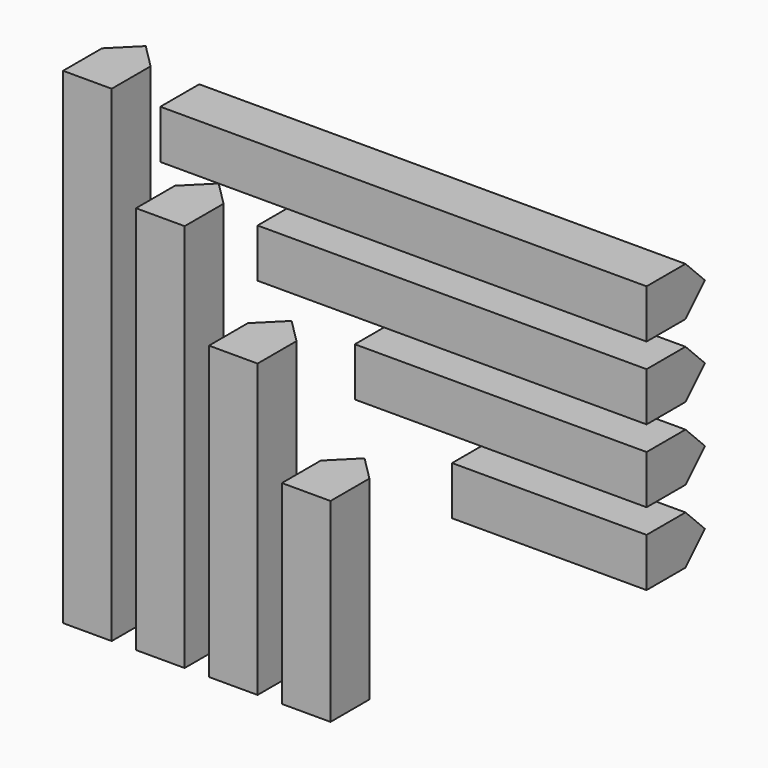
from build123d import *

# Parameters (mm, degrees)
F0_W      = 10
F0_H      = 100
F1_DEPTH  = 15
F0_H_2    = 80
F0_H_3    = 60
F0_H_4    = 40
F0_W_2    = 100
F0_H_5    = 10
F0_W_3    = 80
F0_W_4    = 60
F0_W_5    = 40
F2_SIZE   = 4.99999
F2_2_SIZE = 4.99999
F2_3_SIZE = 4.99999
F2_4_SIZE = 4.99999
F2_5_SIZE = 4.99999
F2_6_SIZE = 4.99999
F2_7_SIZE = 4.99999
F2_8_SIZE = 4.99999


# Not quite as in the source:
# - a fillet or chamfer is up to 0.001 mm smaller than in the source, because OpenCascade refuses the exact size


with BuildPart() as f1:
    # F0 (on Front) → F1 (new body)
    with BuildSketch(Plane.XZ):
        with Locations((-76.6543754238, -0.7175691426)):
            Rectangle(F0_W, F0_H)
    extrude(amount=F1_DEPTH)

    # F2#8 (size 5 in the source; OpenCascade refuses exactly that, so slightly less here)
    f2_8_edges = [f1.edges().sort_by_distance(p)[0] for p in [
        (-71.654375, 0, -0.717569),
        (-81.654375, 0, -0.717569),
    ]]
    chamfer(f2_8_edges, length=F2_8_SIZE)


with BuildPart() as f1b:
    # F0 (on Front) → F1, piece 2 (new body)
    with BuildSketch(Plane.XZ):
        with Locations((-61.6543754238, -10.7175691426)):
            Rectangle(F0_W, F0_H_2)
    extrude(amount=F1_DEPTH)

    # F2#7 (size 5 in the source; OpenCascade refuses exactly that, so slightly less here)
    f2_7_edges = [f1b.edges().sort_by_distance(p)[0] for p in [
        (-56.654375, 0, -10.717569),
        (-66.654375, 0, -10.717569),
    ]]
    chamfer(f2_7_edges, length=F2_7_SIZE)


with BuildPart() as f1c:
    # F0 (on Front) → F1, piece 3 (new body)
    with BuildSketch(Plane.XZ):
        with Locations((-46.6543754238, -20.7175691426)):
            Rectangle(F0_W, F0_H_3)
    extrude(amount=F1_DEPTH)

    # F2#6 (size 5 in the source; OpenCascade refuses exactly that, so slightly less here)
    f2_6_edges = [f1c.edges().sort_by_distance(p)[0] for p in [
        (-41.654375, 0, -20.717569),
        (-51.654375, 0, -20.717569),
    ]]
    chamfer(f2_6_edges, length=F2_6_SIZE)


with BuildPart() as f1d:
    # F0 (on Front) → F1, piece 4 (new body)
    with BuildSketch(Plane.XZ):
        with Locations((-31.6543754238, -30.7175691426)):
            Rectangle(F0_W, F0_H_4)
    extrude(amount=F1_DEPTH)

    # F2#5 (size 5 in the source; OpenCascade refuses exactly that, so slightly less here)
    f2_5_edges = [f1d.edges().sort_by_distance(p)[0] for p in [
        (-26.654375, 0, -30.717569),
        (-36.654375, 0, -30.717569),
    ]]
    chamfer(f2_5_edges, length=F2_5_SIZE)


with BuildPart() as f1e:
    # F0 (on Front) → F1, piece 5 (new body)
    with BuildSketch(Plane.XZ):
        with Locations((-11.6543754238, 44.2824308574)):
            Rectangle(F0_W_2, F0_H_5)
    extrude(amount=F1_DEPTH)

    # F2#4 (size 5 in the source; OpenCascade refuses exactly that, so slightly less here)
    f2_4_edges = [f1e.edges().sort_by_distance(p)[0] for p in [
        (-11.654375, 0, 39.282431),
        (-11.654375, 0, 49.282431),
    ]]
    chamfer(f2_4_edges, length=F2_4_SIZE)


with BuildPart() as f1f:
    # F0 (on Front) → F1, piece 6 (new body)
    with BuildSketch(Plane.XZ):
        with Locations((-1.6543754238, 29.2824308574)):
            Rectangle(F0_W_3, F0_H_5)
    extrude(amount=F1_DEPTH)

    # F2#3 (size 5 in the source; OpenCascade refuses exactly that, so slightly less here)
    f2_3_edges = [f1f.edges().sort_by_distance(p)[0] for p in [
        (-1.654375, 0, 24.282431),
        (-1.654375, 0, 34.282431),
    ]]
    chamfer(f2_3_edges, length=F2_3_SIZE)


with BuildPart() as f1g:
    # F0 (on Front) → F1, piece 7 (new body)
    with BuildSketch(Plane.XZ):
        with Locations((8.3456245762, 14.2824308574)):
            Rectangle(F0_W_4, F0_H_5)
    extrude(amount=F1_DEPTH)

    # F2#2 (size 5 in the source; OpenCascade refuses exactly that, so slightly less here)
    f2_2_edges = [f1g.edges().sort_by_distance(p)[0] for p in [
        (8.345625, 0, 9.282431),
        (8.345625, 0, 19.282431),
    ]]
    chamfer(f2_2_edges, length=F2_2_SIZE)


with BuildPart() as f1h:
    # F0 (on Front) → F1, piece 8 (new body)
    with BuildSketch(Plane.XZ):
        with Locations((18.3456245762, -0.7175691426)):
            Rectangle(F0_W_5, F0_H_5)
    extrude(amount=F1_DEPTH)

    # F2 (size 5 in the source; OpenCascade refuses exactly that, so slightly less here)
    f2_edges = [f1h.edges().sort_by_distance(p)[0] for p in [
        (18.345625, 0, -5.717569),
        (18.345625, 0, 4.282431),
    ]]
    chamfer(f2_edges, length=F2_SIZE)


solid = Compound([f1.part, f1b.part, f1c.part, f1d.part, f1e.part, f1f.part, f1g.part, f1h.part])
